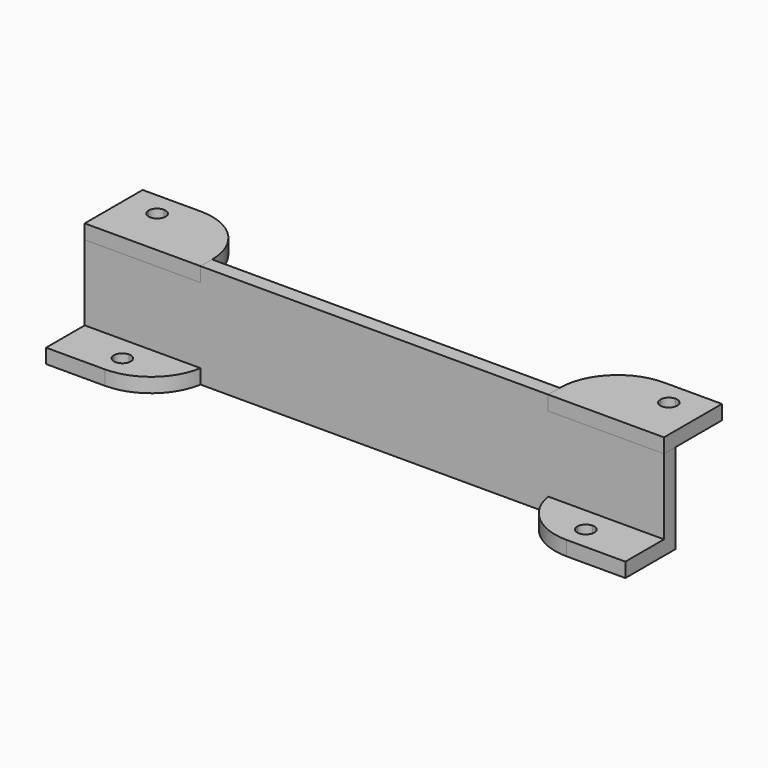
from build123d import *

# Parameters (mm, degrees)
F1_DEPTH    = 3
F0_W        = 12
F0_H        = 3
F2_DEPTH    = 13
F3_T1_DEPTH = 62.160797831
F4_T1_DEPTH = 62.160797831
F5_DEPTH    = 15
F7_R        = 12
F7_2_R      = 12
F9_DEPTH    = 25
F11_DEPTH   = 25


# Not quite as in the source:
# - a fillet or chamfer that OpenCascade refuses, or shapes differently, is made with other operations: its cross-section is extruded or revolved along the edge and cut away or added


with BuildPart() as f1:
    # F0 (on Front) → F1 (new body)
    with BuildSketch(Plane.XZ):
        Polygon((-48, 7.8), (-60, 7.8), (-60, -7.8), (-48, -7.8), (-36, -7.8), (-36, -10.8), (36, -10.8), (36, -7.8), (48, -7.8), (60, -7.8), (60, 7.8), (48, 7.8), (36, 7.8), (36, 10.8), (-36, 10.8), (-36, 7.8), align=None)
    extrude(amount=F1_DEPTH)

    # F0 (on Front) → F2 (join)
    with BuildSketch(Plane.XZ):
        with Locations((-54, -9.3)):
            Rectangle(F0_W, F0_H)
        with Locations((54, -9.3)):
            Rectangle(F0_W, F0_H)
        with Locations((-42, -9.3)):
            Rectangle(F0_W, F0_H)
        with Locations((42, -9.3)):
            Rectangle(F0_W, F0_H)
    extrude(amount=F2_DEPTH)

    # F3: fillet of radius 12 on 1 edges, made by hand

    # F3_s2 → F3_t1 (cut)
    with BuildSketch(Plane.XY.offset(-40.3803989155)):
        with BuildLine():
            ThreePointArc((-36, -3), (-40.0861928738, -10.1651513899), (-47.8321595662, -13))
            Line((-47.8321595662, -13), (-36, -13))
            Line((-36, -13), (-36, -3))
        make_face()
    extrude(amount=F3_T1_DEPTH, mode=Mode.SUBTRACT)

    # F4: fillet of radius 12 on 1 edges, made by hand

    # F4_s2 → F4_t1 (cut)
    with BuildSketch(Plane.XY.offset(-40.3803989155)):
        with BuildLine():
            ThreePointArc((47.8321595662, -13), (40.0861928738, -10.1651513899), (36, -3))
            Line((36, -3), (36, -13))
            Line((36, -13), (47.8321595662, -13))
        make_face()
    extrude(amount=F4_T1_DEPTH, mode=Mode.SUBTRACT)


with BuildPart() as f5:
    # F0 (on Front) → F5 (new body)
    with BuildSketch(Plane.XZ):
        with Locations((-54, 9.3)):
            Rectangle(F0_W, F0_H)
        with Locations((-42, 9.3)):
            Rectangle(F0_W, F0_H)
    extrude(amount=-F5_DEPTH)


with BuildPart() as f5b:
    # F0 (on Front) → F5, piece 2 (new body)
    with BuildSketch(Plane.XZ):
        with Locations((42, 9.3)):
            Rectangle(F0_W, F0_H)
        with Locations((54, 9.3)):
            Rectangle(F0_W, F0_H)
    extrude(amount=-F5_DEPTH)


with BuildPart() as f5_1:
    # F6: moved
    add(f5.part.moved(Location((0, -3, 0))))

    # F7
    f7_edges = [f5_1.edges().sort_by_distance(p)[0] for p in [
        (-36, 12, 9.3),
    ]]
    fillet(f7_edges, radius=F7_R)


with BuildPart() as f5b_1:
    # F6: moved
    add(f5b.part.moved(Location((0, -3, 0))))

    # F7#2
    f7_2_edges = [f5b_1.edges().sort_by_distance(p)[0] for p in [
        (36, 12, 9.3),
    ]]
    fillet(f7_2_edges, radius=F7_2_R)


with BuildPart() as f9:
    # F8 (on Top) → F9 (new body)
    with BuildSketch(Plane.XY):
        with BuildLine():
            ThreePointArc((-53, 8.75), (-54.2374368671, 8.2374368671), (-54.75, 7))
            Line((-54.75, 7), (-53, 7))
            Line((-53, 7), (-53, 8.75))
        make_face()
        with BuildLine():
            Line((-53, 8.75), (-53, 7))
            Line((-53, 7), (-51.25, 7))
            ThreePointArc((-51.25, 7), (-51.7625631329, 8.2374368671), (-53, 8.75))
        make_face()
        with BuildLine():
            Line((-53, 7), (-53, 5.25))
            ThreePointArc((-53, 5.25), (-51.7625631329, 5.7625631329), (-51.25, 7))
            Line((-51.25, 7), (-53, 7))
        make_face()
        with BuildLine():
            ThreePointArc((-54.75, 7), (-54.2374368671, 5.7625631329), (-53, 5.25))
            Line((-53, 5.25), (-53, 7))
            Line((-53, 7), (-54.75, 7))
        make_face()
    extrude(amount=F9_DEPTH)


with BuildPart() as f9b:
    # F8 (on Top) → F9, piece 2 (new body)
    with BuildSketch(Plane.XY):
        with BuildLine():
            ThreePointArc((51.25, 7), (51.7625631329, 5.7625631329), (53, 5.25))
            Line((53, 5.25), (53, 7))
            Line((53, 7), (51.25, 7))
        make_face()
        with BuildLine():
            Line((53, 7), (53, 5.25))
            ThreePointArc((53, 5.25), (54.2374368671, 5.7625631329), (54.75, 7))
            Line((54.75, 7), (53, 7))
        make_face()
        with BuildLine():
            Line((53, 8.75), (53, 7))
            Line((53, 7), (54.75, 7))
            ThreePointArc((54.75, 7), (54.2374368671, 8.2374368671), (53, 8.75))
        make_face()
        with BuildLine():
            Line((51.25, 7), (53, 7))
            Line((53, 7), (53, 8.75))
            ThreePointArc((53, 8.75), (51.7625631329, 8.2374368671), (51.25, 7))
        make_face()
    extrude(amount=F9_DEPTH)


with BuildPart() as f5_2:
    add(f5_1.part)

    # F10: cut F9, F9b
    add(f9.part, mode=Mode.SUBTRACT)
    add(f9b.part, mode=Mode.SUBTRACT)


with BuildPart() as f5b_2:
    add(f5b_1.part)

    # F10: cut F9, F9b
    add(f9.part, mode=Mode.SUBTRACT)
    add(f9b.part, mode=Mode.SUBTRACT)


with BuildPart() as f11:
    # F8 (on Top) → F11 (new body)
    with BuildSketch(Plane.XY):
        with BuildLine():
            ThreePointArc((-46.274432838, -8.2105052471), (-46.7869959709, -6.97306838), (-48.024432838, -6.4605052471))
            Line((-48.024432838, -6.4605052471), (-48.024432838, -8.2105052471))
            Line((-48.024432838, -8.2105052471), (-46.274432838, -8.2105052471))
        make_face()
        with BuildLine():
            Line((-48.024432838, -8.2105052471), (-48.024432838, -6.4605052471))
            ThreePointArc((-48.024432838, -6.4605052471), (-49.261869705, -6.97306838), (-49.774432838, -8.2105052471))
            Line((-49.774432838, -8.2105052471), (-48.024432838, -8.2105052471))
        make_face()
        with BuildLine():
            Line((-48.024432838, -8.2105052471), (-49.774432838, -8.2105052471))
            ThreePointArc((-49.774432838, -8.2105052471), (-49.261869705, -9.4479421142), (-48.024432838, -9.9605052471))
            Line((-48.024432838, -9.9605052471), (-48.024432838, -8.2105052471))
        make_face()
        with BuildLine():
            Line((-46.274432838, -8.2105052471), (-48.024432838, -8.2105052471))
            Line((-48.024432838, -8.2105052471), (-48.024432838, -9.9605052471))
            ThreePointArc((-48.024432838, -9.9605052471), (-46.7869959709, -9.4479421142), (-46.274432838, -8.2105052471))
        make_face()
    extrude(amount=-F11_DEPTH)


with BuildPart() as f11b:
    # F8 (on Top) → F11, piece 2 (new body)
    with BuildSketch(Plane.XY):
        with BuildLine():
            ThreePointArc((49.725567162, -8.2105052471), (49.2130040291, -6.97306838), (47.975567162, -6.4605052471))
            Line((47.975567162, -6.4605052471), (47.975567162, -8.2105052471))
            Line((47.975567162, -8.2105052471), (49.725567162, -8.2105052471))
        make_face()
        with BuildLine():
            Line((47.975567162, -8.2105052471), (47.975567162, -6.4605052471))
            ThreePointArc((47.975567162, -6.4605052471), (46.738130295, -6.97306838), (46.225567162, -8.2105052471))
            Line((46.225567162, -8.2105052471), (47.975567162, -8.2105052471))
        make_face()
        with BuildLine():
            Line((47.975567162, -9.9605052471), (47.975567162, -8.2105052471))
            Line((47.975567162, -8.2105052471), (46.225567162, -8.2105052471))
            ThreePointArc((46.225567162, -8.2105052471), (46.738130295, -9.4479421142), (47.975567162, -9.9605052471))
        make_face()
        with BuildLine():
            Line((49.725567162, -8.2105052471), (47.975567162, -8.2105052471))
            Line((47.975567162, -8.2105052471), (47.975567162, -9.9605052471))
            ThreePointArc((47.975567162, -9.9605052471), (49.2130040291, -9.4479421142), (49.725567162, -8.2105052471))
        make_face()
    extrude(amount=-F11_DEPTH)


with BuildPart() as f1_1:
    add(f1.part)

    # F12: cut F11, F11b
    add(f11.part, mode=Mode.SUBTRACT)
    add(f11b.part, mode=Mode.SUBTRACT)


solid = Compound([f5_2.part, f5b_2.part, f1_1.part])
